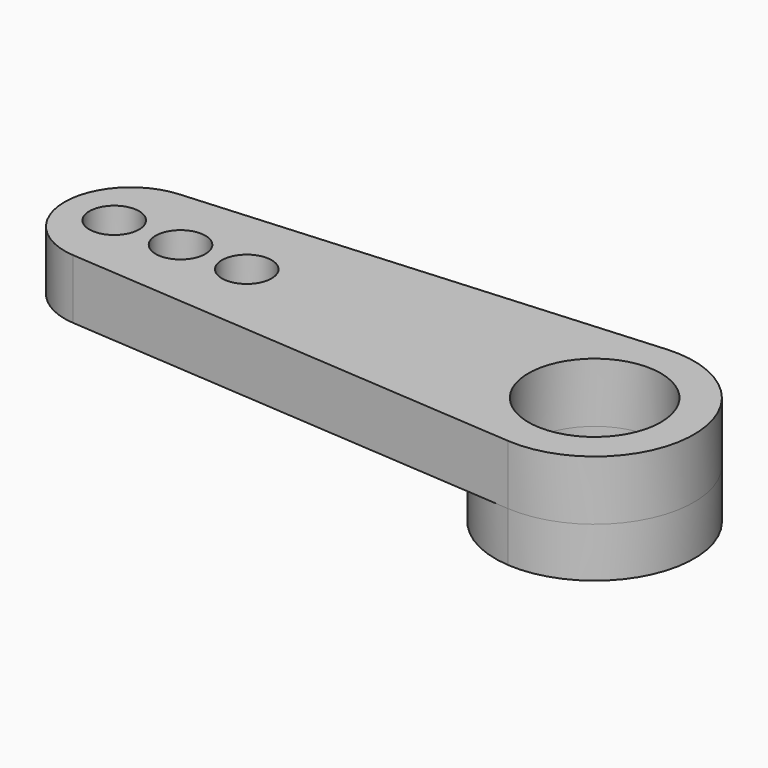
from build123d import *
from build123d import SkipClean  # not in build123d's __all__

# Parameters (mm, degrees)
F0_R     = 0.75
F0_R_2   = 2
F1_DEPTH = 1.8
F2_R     = 2
F3_DEPTH = 1.5


with BuildPart() as f1:
    # F0 (on Top) → F1 (new body)
    with BuildSketch(Plane.XY):
        with BuildLine():
            Line((-14.1428571429, -1.9948914348), (-0.2142857143, -2.9923371522))
            ThreePointArc((-0.2142857143, -2.9923371522), (3, 0), (-0.2142857143, 2.9923371522))
            Line((-0.2142857143, 2.9923371522), (-14.1428571429, 1.9948914348))
            ThreePointArc((-14.1428571429, 1.9948914348), (-16, 0), (-14.1428571429, -1.9948914348))
        make_face()
        with Locations((-14.5, 0)):
            Circle(F0_R, mode=Mode.SUBTRACT)
        with Locations((-12.5, 0)):
            Circle(F0_R, mode=Mode.SUBTRACT)
        with Locations((-10.5, 0)):
            Circle(F0_R, mode=Mode.SUBTRACT)
        Circle(F0_R_2, mode=Mode.SUBTRACT)
    extrude(amount=F1_DEPTH)

    # F2 (on face) → F3 (join)
    with BuildSketch(Plane(origin=(0, 0, 0), x_dir=(1, 0, 0), z_dir=(0, 0, -1))):
        with BuildLine():
            ThreePointArc((-0.2142857143, -2.9923371522), (3, 0), (-0.2142857143, 2.9923371522))
            ThreePointArc((-0.2142857143, 2.9923371522), (-3, 0), (-0.2142857143, -2.9923371522))
        make_face()
        Circle(F2_R, mode=Mode.SUBTRACT)
    with SkipClean():  # cleaning this boolean's faces spoils the solid; the shape is the same uncleaned
        extrude(amount=F3_DEPTH)


solid = f1.part
